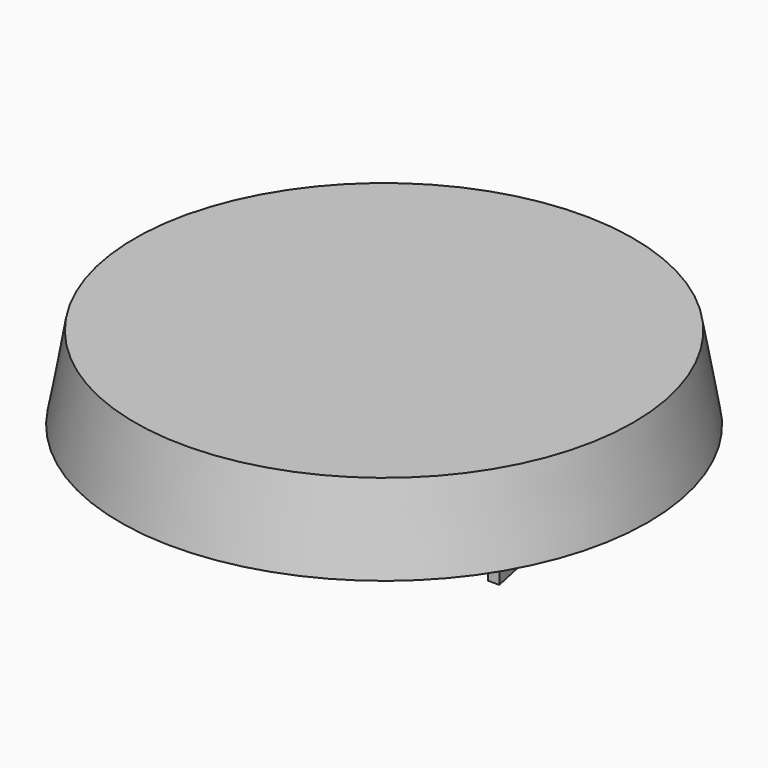
from build123d import *

# Parameters (mm, degrees)
F0_R           = 30
F1_DEPTH       = 10
F1_TAPER       = -10
F2_TEXT_SIZE   = 16.8922161436
F2_TEXT_SIZE_2 = 10.3927492447
F2_TEXT_SIZE_3 = 17.6692821854
F3_DEPTH       = 2


# Not quite as in the source:
# - Text() gives the source's letters only with a copy of the font that has no kerning and outlines rounded to 1/6400 em; it was checked with that copy


with BuildPart() as f1:
    # F0 (on Top) → F1 (new body)
    with BuildSketch(Plane.XY):
        Circle(F0_R)
    extrude(amount=-F1_DEPTH, taper=F1_TAPER)

    # F2 (on face) → F3 (join)
    with BuildSketch(Plane(origin=(0, 0, -10), x_dir=(1, 0, 0), z_dir=(0, 0, -1))):
        with Locations((-27.5, 2.8376043766)):
            Text('God Jul', F2_TEXT_SIZE, font='Open Sans', font_style=FontStyle.ITALIC, text_align=(TextAlign.LEFT, TextAlign.BOTTOM))
        with Locations((-26, -11.7218831735)):
            Text('fam.', F2_TEXT_SIZE_2, font='Open Sans', font_style=FontStyle.ITALIC, text_align=(TextAlign.LEFT, TextAlign.BOTTOM))
        with Locations((-8, -11.7218831735)):
            Text('Gren', F2_TEXT_SIZE_3, font='Open Sans', font_style=FontStyle.ITALIC, text_align=(TextAlign.LEFT, TextAlign.BOTTOM))
    extrude(amount=F3_DEPTH)


solid = f1.part
